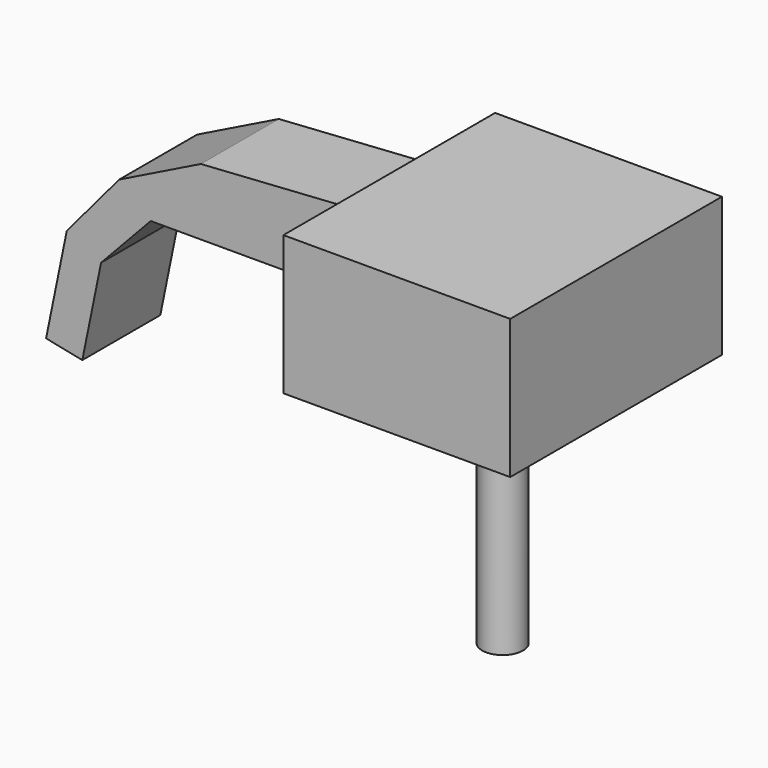
from build123d import *

# Parameters (mm, degrees)
F0_R     = 1.85928
F1_DEPTH = 21.59
F2_R     = 1.07823
F3_DEPTH = 3.175
F4_W     = 20.6828571429
F4_H     = 24.13
F5_DEPTH = 12.7
F7_DEPTH = 4.445


# Not quite as in the source:
# - a feature names something its author has since deleted; it is built from what else it names


with BuildPart() as f1:
    # F0 (on Top) → F1 (new body)
    with BuildSketch(Plane.XY):
        Circle(F0_R)
    extrude(amount=-F1_DEPTH)

    # F2 (on Front) → F3 (cut, symmetric)
    with BuildSketch(Plane.XZ):
        with Locations((0, -2.7295311447)):
            Circle(F2_R)
    extrude(amount=F3_DEPTH, both=True, mode=Mode.SUBTRACT)

    # F4 (on Top) → F5 (join)
    with BuildSketch(Plane.XY):
        Rectangle(F4_W, F4_H)
    extrude(amount=F5_DEPTH)

    # F6 (on Front) → F7 (join, symmetric)
    with BuildSketch(Plane.XZ):
        Polygon((-9.8489131778, 4.8180790618), (-10.3458696976, 11.7754703388), (-23.9624772221, 10.8809489757), (-31.4168259501, 7.2034704499), (-36.187607795, 1.5381660778), (-38.076043129, -7.7052260749), (-34.7716075912, -8.3803259436), (-33.0594976471, 0), (-28.5344794393, 4.8180790618), (-21.7758696526, 4.8180790618), align=None)
    extrude(amount=F7_DEPTH, both=True)


solid = f1.part
